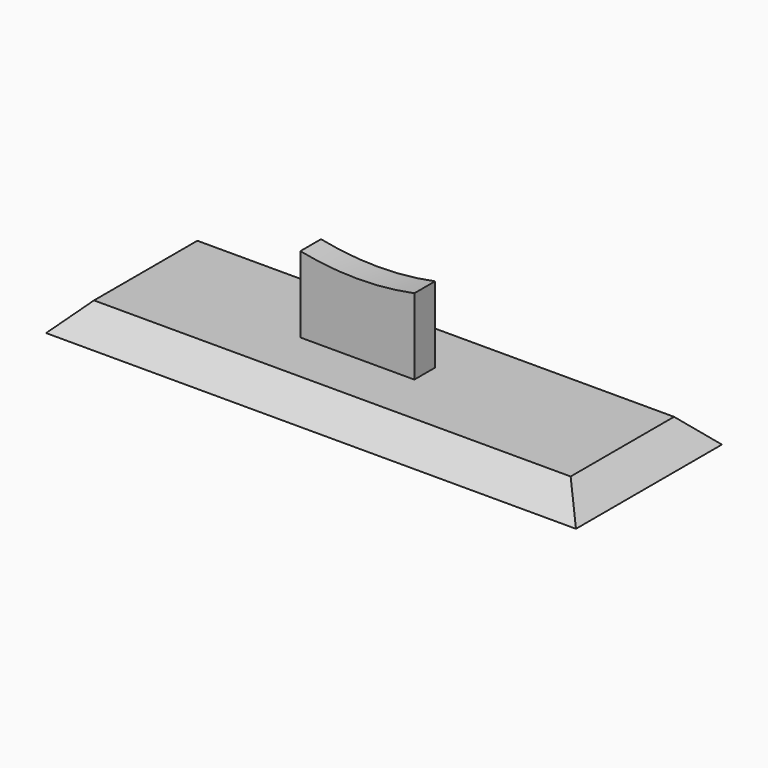
from build123d import *

# Parameters (mm, degrees)
F0_W        = 70.7058645785
F0_H        = 25
F1_DEPTH    = 3.5
F2_T1_DEPTH = 91.2793284822
F2_T3_DEPTH = 45.5734639037
F3_W        = 8
F3_H        = 3.4
F4_DEPTH    = 3.5
F6_DEPTH    = 1.7


# Not quite as in the source:
# - a fillet or chamfer that OpenCascade refuses, or shapes differently, is made with other operations: its cross-section is extruded or revolved along the edge and cut away or added


with BuildPart() as f1:
    # F0 (on Top) → F1 (new body)
    with BuildSketch(Plane.XY):
        with Locations((2.1470677108, 0)):
            Rectangle(F0_W, F0_H)
    extrude(amount=F1_DEPTH)

    # F2: chamfer of 4 on 4 edges, made by hand

    # F2_s2 → F2_t1 (cut)
    with BuildSketch(Plane.YZ.offset(-43.4925965303)):
        Polygon((-12.5, -0.5), (-8.5, 3.5), (-12.5, 3.5), align=None)
        Polygon((12.5, -0.5), (8.5, 3.5), (12.5, 3.5), align=None)
    extrude(amount=F2_T1_DEPTH, mode=Mode.SUBTRACT)

    # F2_s4 → F2_t3 (cut)
    with BuildSketch(Plane.XZ.offset(-22.7867319519)):
        Polygon((-33.2058645785, -0.5), (-29.2058645785, 3.5), (-33.2058645785, 3.5), align=None)
        Polygon((37.5, -0.5), (33.5, 3.5), (37.5, 3.5), align=None)
    extrude(amount=F2_T3_DEPTH, mode=Mode.SUBTRACT)

    # F3 (on Top) → F4 (cut)
    with BuildSketch(Plane.XY):
        Rectangle(F3_W, F3_H)
    extrude(amount=F4_DEPTH, mode=Mode.SUBTRACT)


with BuildPart() as f6:
    # F5 (on Front) → F6 (new body, symmetric)
    with BuildSketch(Plane.XZ):
        with BuildLine():
            Line((-4, 3.5), (-4, 0))
            Line((-4, 0), (4, 0))
            Line((4, 0), (4, 3.5))
            Line((4, 3.5), (7.5, 3.5))
            Line((7.5, 3.5), (7.5, 13.5))
            ThreePointArc((7.5, 13.5), (0, 12.7423461417), (-7.5, 13.5))
            Line((-7.5, 13.5), (-7.5, 3.5))
            Line((-7.5, 3.5), (-4, 3.5))
        make_face()
    extrude(amount=F6_DEPTH, both=True)


solid = Compound([f1.part, f6.part])
